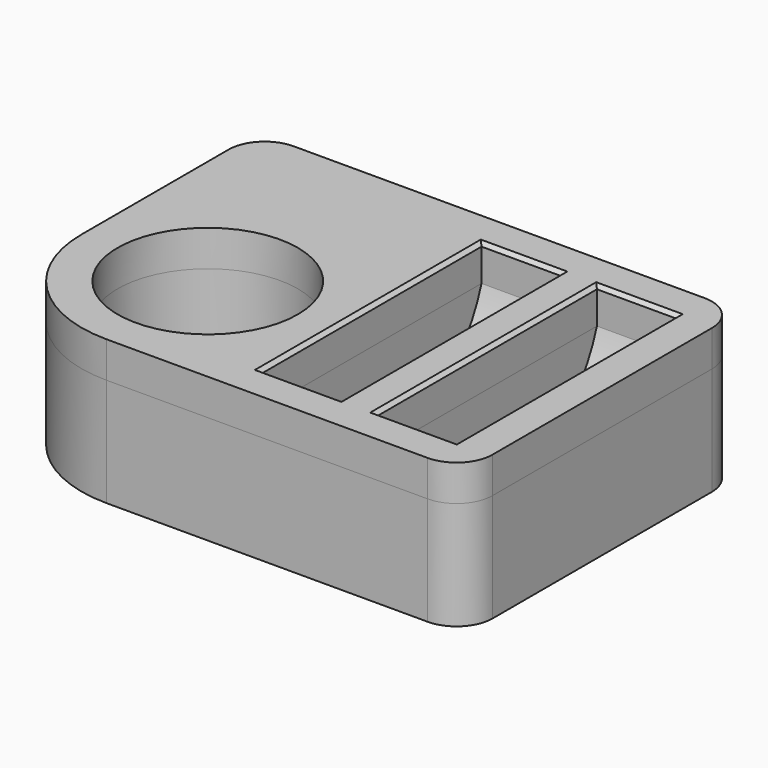
from build123d import *

# Parameters (mm, degrees)
F0_R         = 12.5
F1_DEPTH     = 21
F2_W         = 11
F2_H         = 20
F4_W         = 83.8048234582
F4_H         = 10.6309341639
F5_DEPTH     = 48.001
F6_TEXT_SIZE = 8.3333333333
F7_DEPTH     = 1
F8_R         = 12.5
F8_W         = 11
F8_H         = 38.1575680567
F9_DEPTH     = 5
F10_SIZE     = 0.5


# Not quite as in the source:
# - Text() gives the source's letters only with a copy of the font that has no kerning and outlines rounded to 1/6400 em; it was checked with that copy


with BuildPart() as f1:
    # F0 (on Top) → F1 (new body)
    with BuildSketch(Plane.XY):
        with BuildLine():
            ThreePointArc((0, 17.5), (5.1256313292, 5.1256313292), (17.5, 0))
            Line((17.5, 0), (62, 0))
            ThreePointArc((62, 0), (65.5355339059, 1.4644660941), (67, 5))
            Line((67, 5), (67, 43))
            ThreePointArc((67, 43), (65.5355339059, 46.5355339059), (62, 48))
            Line((62, 48), (5, 48))
            ThreePointArc((5, 48), (1.4644660941, 46.5355339059), (0, 43))
            Line((0, 43), (0, 17.5))
        make_face()
        with Locations((17.5, 17.5)):
            Circle(F0_R, mode=Mode.SUBTRACT)
    extrude(amount=F1_DEPTH)

    # F2 (on face) → F3 (revolve, cut)
    with BuildSketch(Plane.XY.offset(21)):
        with Locations((40.5, 14)):
            Rectangle(F2_W, F2_H)
        with Locations((56.5, 14)):
            Rectangle(F2_W, F2_H)
    revolve(axis=Axis((40.5, 24, 21), (1, 0, 0)), mode=Mode.SUBTRACT)

    # F4 (on face) → F5 (cut, through all)
    with BuildSketch(Plane.XZ):
        with Locations((41.9024117291, 20.315467082)):
            Rectangle(F4_W, F4_H)
    extrude(amount=-F5_DEPTH, mode=Mode.SUBTRACT)

    # F6 (on face) → F7 (cut)
    with BuildSketch(Plane(origin=(0, 0, 0), x_dir=(1, 0, 0), z_dir=(0, 0, -1))):
        with Locations((30, -11)):
            Text('928', F6_TEXT_SIZE, font='Open Sans', text_align=(TextAlign.LEFT, TextAlign.BOTTOM))
    extrude(amount=-F7_DEPTH, mode=Mode.SUBTRACT)


with BuildPart() as f9:
    # F8 (on face) → F9 (new body)
    with BuildSketch(Plane.XY.offset(15)):
        with BuildLine():
            ThreePointArc((0, 17.5), (5.1256313292, 5.1256313292), (17.5, 0))
            Line((17.5, 0), (62, 0))
            ThreePointArc((62, 0), (65.5355339059, 1.4644660941), (67, 5))
            Line((67, 5), (67, 43))
            ThreePointArc((67, 43), (65.5355339059, 46.5355339059), (62, 48))
            Line((62, 48), (5, 48))
            ThreePointArc((5, 48), (1.4644660941, 46.5355339059), (0, 43))
            Line((0, 43), (0, 17.5))
        make_face()
        with Locations((17.5, 17.5)):
            Circle(F8_R, mode=Mode.SUBTRACT)
        with Locations((40.5, 24)):
            Rectangle(F8_W, F8_H, mode=Mode.SUBTRACT)
        with Locations((56.5, 24)):
            Rectangle(F8_W, F8_H, mode=Mode.SUBTRACT)
    extrude(amount=F9_DEPTH)

    # F10
    f10_edges = [f9.edges().sort_by_distance(p)[0] for p in [
        (62, 24, 20),
        (56.5, 4.921216, 20),
        (51, 24, 20),
        (40.5, 4.921216, 20),
        (35, 24, 20),
        (46, 24, 20),
        (40.5, 43.078784, 20),
        (56.5, 43.078784, 20),
    ]]
    chamfer(f10_edges, length=F10_SIZE)


solid = Compound([f1.part, f9.part])
